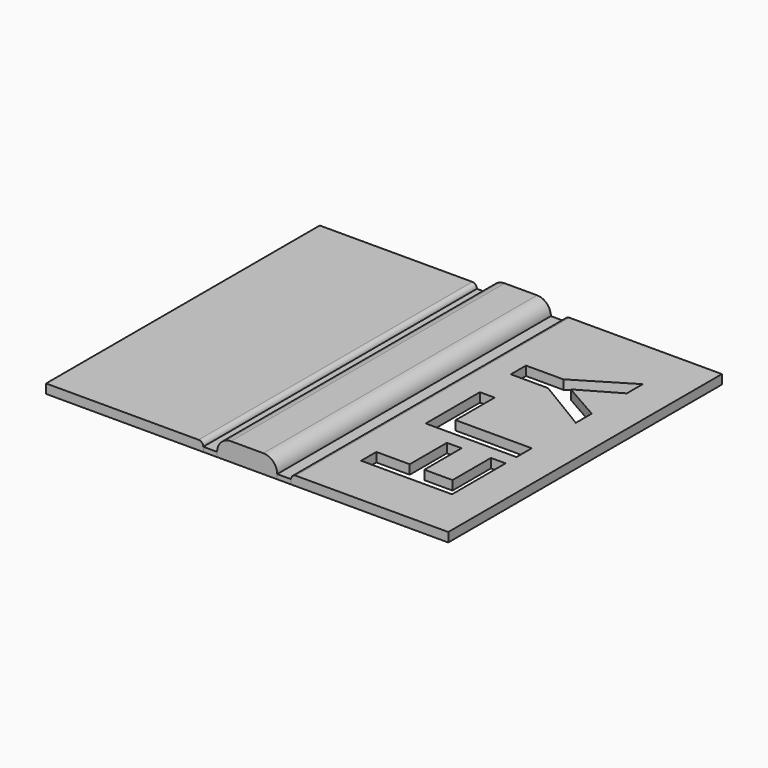
from build123d import *

# Parameters (mm, degrees)
F0_W         = 17
F0_H         = 37
F1_DEPTH     = 1
F0_W_2       = 6.5
F2_DEPTH     = 2
F0_W_3       = 1.5
F3_DEPTH     = 0.5
F4_R         = 1.5
F5_R         = 0.5
F5_2_R       = 0.5
F6_TEXT_SIZE = 14.2858394257
F7_DEPTH     = 25


# Not quite as in the source:
# - Text() gives the source's letters only with a copy of the font that has no kerning and outlines rounded to 1/6400 em; it was checked with that copy


with BuildPart() as f1:
    # F0 (on Top) → F1 (new body)
    with BuildSketch(Plane.XY):
        Rectangle(F0_W, F0_H)
    extrude(amount=F1_DEPTH)

    # F5#2
    f5_2_edges = [f1.edges().sort_by_distance(p)[0] for p in [
        (-8.5, 0, 1),
    ]]
    fillet(f5_2_edges, radius=F5_2_R)

    # F6 (on face) → F7 (cut)
    with BuildSketch(Plane(origin=(0, 0, 0), x_dir=(1, 0, 0), z_dir=(0, 0, -1))):
        with Locations(Location((-5.3916570707, 13.8706572174), (0, 0, -90))):
            Text('FLY', F6_TEXT_SIZE, font='Arimo', font_style=FontStyle.BOLD, text_align=(TextAlign.LEFT, TextAlign.BOTTOM))
    extrude(amount=-F7_DEPTH, mode=Mode.SUBTRACT)


with BuildPart() as f1b:
    # F0 (on Top) → F1, piece 2 (new body)
    with BuildSketch(Plane.XY):
        with Locations((-26.5, 0)):
            Rectangle(F0_W, F0_H)
    extrude(amount=F1_DEPTH)

    # F5
    f5_edges = [f1b.edges().sort_by_distance(p)[0] for p in [
        (-18, 0, 1),
    ]]
    fillet(f5_edges, radius=F5_R)


with BuildPart() as f2:
    # F0 (on Top) → F2 (new body)
    with BuildSketch(Plane.XY):
        with Locations((-13.25, 0)):
            Rectangle(F0_W_2, F0_H)
    extrude(amount=F2_DEPTH)

    # F4
    f4_edges = [f2.edges().sort_by_distance(p)[0] for p in [
        (-10, 0, 2),
        (-16.5, 0, 2),
    ]]
    fillet(f4_edges, radius=F4_R)


with BuildPart() as f3:
    # F0 (on Top) → F3 (new body)
    with BuildSketch(Plane.XY):
        with Locations((-17.25, 0)):
            Rectangle(F0_W_3, F0_H)
    extrude(amount=F3_DEPTH)


with BuildPart() as f3b:
    # F0 (on Top) → F3, piece 2 (new body)
    with BuildSketch(Plane.XY):
        with Locations((-9.25, 0)):
            Rectangle(F0_W_3, F0_H)
    extrude(amount=F3_DEPTH)


solid = Compound([f1.part, f1b.part, f2.part, f3.part, f3b.part])
